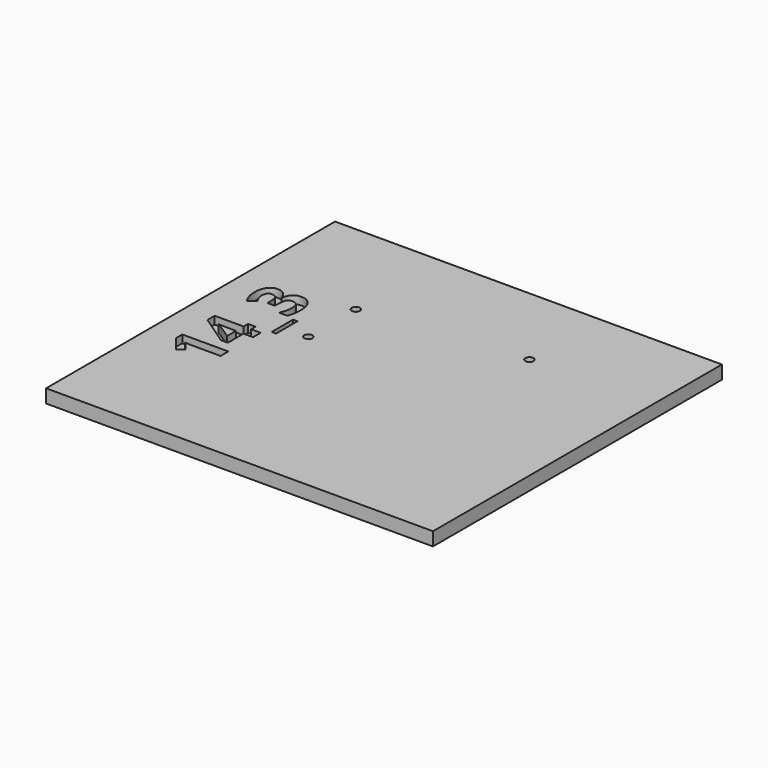
from build123d import *

# Parameters (mm, degrees)
F0_W         = 75
F0_H         = 70
F1_DEPTH     = 2.6
F2_TEXT_SIZE = 12.5
F3_DEPTH     = 1.5
F4_R         = 0.8
F5_DEPTH     = 2.6


# Not quite as in the source:
# - Text() gives the source's letters only with a copy of the font that has no kerning and outlines rounded to 1/6400 em; it was checked with that copy


with BuildPart() as f1:
    # F0 (on Top) → F1 (new body)
    with BuildSketch(Plane.XY):
        with Locations((-5.6587231159, 13.3350909071)):
            Rectangle(F0_W, F0_H)
    extrude(amount=F1_DEPTH)

    # F2 (on face) → F3 (cut)
    with BuildSketch(Plane.XY.offset(2.6)):
        with Locations(Location((-29.1587231159, -0.1649090929), (0, 0, 90))):
            Text('14_3', F2_TEXT_SIZE, font='Open Sans', font_style=FontStyle.BOLD, text_align=(TextAlign.LEFT, TextAlign.BOTTOM))
    extrude(amount=-F3_DEPTH, mode=Mode.SUBTRACT)

    # F4 (on face) → F5 (cut, through all)
    with BuildSketch(Plane.XY.offset(2.6)):
        with BuildLine():
            ThreePointArc((-23.1587231159, 16.9965287348), (-23.5087231159, 16.3350909071), (-23.1587231159, 15.6736530793))
            Line((-23.1587231159, 15.6736530793), (-23.1587231159, 16.9965287348))
        make_face()
        with BuildLine():
            Line((-23.1587231159, 16.9965287348), (-23.1587231159, 15.6736530793))
            ThreePointArc((-23.1587231159, 15.6736530793), (-22.3345573772, 15.6279841259), (-21.9087231159, 16.3350909071))
            ThreePointArc((-21.9087231159, 16.3350909071), (-22.3345573772, 17.0421976882), (-23.1587231159, 16.9965287348))
        make_face()
        with BuildLine():
            ThreePointArc((-23.1587231159, 28.4965287348), (-23.5087231159, 27.8350909071), (-23.1587231159, 27.1736530793))
            Line((-23.1587231159, 27.1736530793), (-23.1587231159, 28.4965287348))
        make_face()
        with BuildLine():
            Line((-23.1587231159, 28.4965287348), (-23.1587231159, 27.1736530793))
            ThreePointArc((-23.1587231159, 27.1736530793), (-22.3345573772, 27.1279841259), (-21.9087231159, 27.8350909071))
            ThreePointArc((-21.9087231159, 27.8350909071), (-22.3345573772, 28.5421976882), (-23.1587231159, 28.4965287348))
        make_face()
        with Locations((8.0912768841, 31.3850909071)):
            Circle(F4_R)
    extrude(amount=-F5_DEPTH, mode=Mode.SUBTRACT)


solid = f1.part
